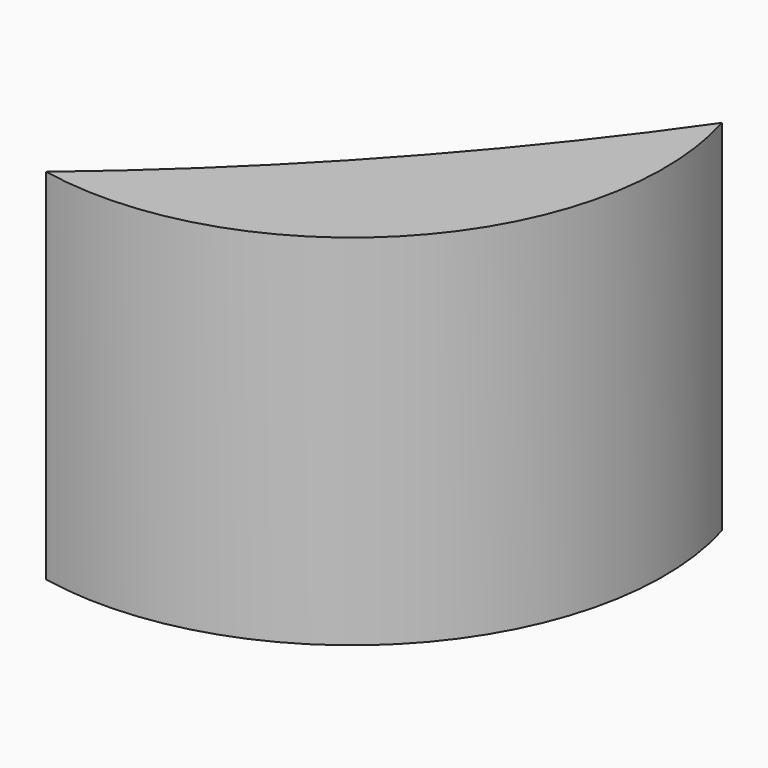
from build123d import *

# Parameters (mm, degrees)
F1_DEPTH = 9.398


# Not quite as in the source:
# - a feature names something its author has since deleted; it is built from what else it names


with BuildPart() as f1:
    # F0 (on Top) → F1 (new body)
    with BuildSketch(Plane.XY):
        with BuildLine():
            ThreePointArc((14.3654148349, 24.020783957), (9.9874199255, 18.5472363603), (4.9292104318, 13.6953213324))
            ThreePointArc((4.9292104318, 13.6953213324), (12.5618804591, 16.1944956933), (14.3654148349, 24.020783957))
        make_face()
    extrude(amount=F1_DEPTH)


solid = f1.part
